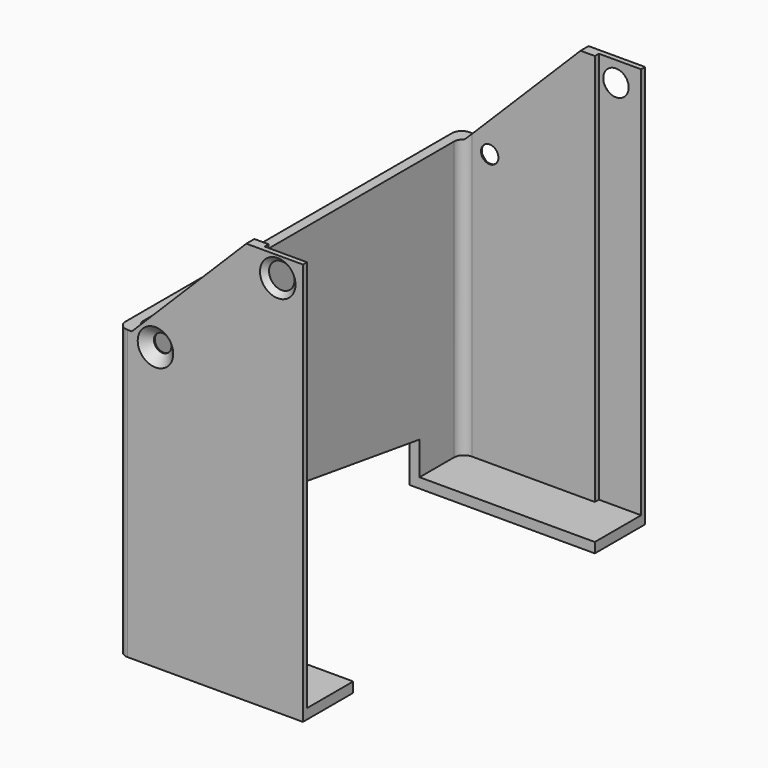
from build123d import *

# Parameters (mm, degrees)
F1_DEPTH       = 107.95
F2_T           = 2.54
F4_R           = 2.54
F3_W           = 32.7291795984
F3_H           = 105.41
F5_DEPTH       = 99.06
F7_D           = 4.4
F7_DEPTH       = 37.1856
F7_CSINK_D     = 8.96
F7_CSINK_ANGLE = 90
F7_TIP         = 1.3218933619
F9_D           = 4.4
F9_DEPTH       = 37.1856
F9_CSINK_D     = 8.96
F9_CSINK_ANGLE = 90
F9_TIP         = 1.3218933619
F10_W          = 76.2
F10_H          = 10.922
F11_DEPTH      = 56.134
F12_TEXT_SIZE  = 17.6388888889
F13_DEPTH      = 0.5334
F14_W          = 15.1848194814
F14_H          = 102.87
F15_DEPTH      = 70.1687200073
F16_DEPTH      = 70.1687200073
F17_R          = 2.54


# Not quite as in the source:
# - a shell that OpenCascade refuses in one call is made with other operations: the cavity is built on its own and cut out
# - a feature names something its author has since deleted; it is built from what else it names
# - Text() gives the source's letters only with a copy of the font that has no kerning and outlines rounded to 1/6400 em; it was checked with that copy


with BuildPart() as f1:
    # F0 (on Front) → F1 (new body)
    with BuildSketch(Plane.XZ):
        Polygon((0, 0), (0, 101.6), (-14.27734, 101.6), (-43.1686199927, 72.7087200073), (-46.7614, 72.7087200073), (-46.7614, 0), align=None)
    extrude(amount=F1_DEPTH)

    # F2: shell of thickness 2.54, made by hand


with BuildPart() as f2_core1:
    # F2_t2: copy of F1
    add(f1.part)

    # the walls: a layer under each face that stays
    f2_faces = [f2_core1.faces().sort_by_distance(p)[0] for p in [
        (-44.9650099964, -53.975, 72.7087200073),
        (-46.7614, -53.975, 36.3543600036),
        (-23.3807, -53.975, 0),
        (-23.3807, 0, 50.8),
        (-23.3807, -107.95, 50.8),
    ]]
    thicken(f2_faces, amount=-F2_T, mode=Mode.SUBTRACT)


with BuildPart() as f1_1:
    add(f1.part)

    # what is left inside the walls is the cavity
    f2_cavity = [f2_core1.part.solids().sort_by_distance(p)[0] for p in [
        (-0.0254, -71.12, 52.07),
    ]]
    add(f2_cavity, mode=Mode.SUBTRACT)

    # F4
    f4_edges = [f1_1.edges().sort_by_distance(p)[0] for p in [
        (-46.7614, -107.95, 36.35436),
        (-46.7614, 0, 36.35436),
    ]]
    fillet(f4_edges, radius=F4_R)

    # F3 (on face) → F5 (cut, through all)
    with BuildSketch(Plane.XY.offset(101.6)):
        with Locations((5.6965897992, -53.975)):
            Rectangle(F3_W, F3_H)
    extrude(amount=-F5_DEPTH, mode=Mode.SUBTRACT)

    # F7
    with Locations(Plane.XZ.offset(107.95)):
        with Locations((-37.20084, 71.12), (-6.35, 96.52)):
            CounterSinkHole(F7_D / 2, F7_CSINK_D / 2, depth=F7_DEPTH, counter_sink_angle=F7_CSINK_ANGLE)
            with Locations((0, 0, -(F7_DEPTH + F7_TIP / 2))):  # 118° drill point
                Cone(0, F7_D / 2, F7_TIP, mode=Mode.SUBTRACT)

    # F9
    with Locations(Plane(origin=(0, 0, 0), x_dir=(-1, 0, 0), z_dir=(0, 1, 0))):
        with Locations((37.20084, 71.12), (6.35, 96.52)):
            CounterSinkHole(F9_D / 2, F9_CSINK_D / 2, depth=F9_DEPTH, counter_sink_angle=F9_CSINK_ANGLE)
            with Locations((0, 0, -(F9_DEPTH + F9_TIP / 2))):  # 118° drill point
                Cone(0, F9_D / 2, F9_TIP, mode=Mode.SUBTRACT)

    # F10 (on face) → F11 (cut)
    with BuildSketch(Plane(origin=(-46.7614, 0, 0), x_dir=(0, -1, 0), z_dir=(-1, 0, 0))):
        Polygon((53.975, 16.51), (15.875, 10.922), (92.075, 10.922), align=None)
        with Locations((53.975, 5.461)):
            Rectangle(F10_W, F10_H)
    extrude(amount=-F11_DEPTH, mode=Mode.SUBTRACT)

    # F12 (on face) → F13 (cut)
    with BuildSketch(Plane(origin=(-46.7614, 0, 0), x_dir=(0, -1, 0), z_dir=(-1, 0, 0))):
        with Locations((36.2382703993, 53.6587200073)):
            Text('THC', F12_TEXT_SIZE, font='Open Sans', font_style=FontStyle.BOLD, text_align=(TextAlign.LEFT, TextAlign.BOTTOM))
        with Locations((12.3155273438, 38.4187200073)):
            Text('MACHINES', F12_TEXT_SIZE, font='Open Sans', font_style=FontStyle.ITALIC, text_align=(TextAlign.LEFT, TextAlign.BOTTOM))
    extrude(amount=-F13_DEPTH, mode=Mode.SUBTRACT)

    # F14 (on face) → F15 (cut, through all)
    with BuildSketch(Plane.XY.offset(72.7087200073)):
        with Locations((-36.6289902593, -53.975)):
            Rectangle(F14_W, F14_H)
    extrude(amount=-F15_DEPTH, mode=Mode.SUBTRACT)

    # F14 (on face) → F16 (cut, through all)
    with BuildSketch(Plane.XY.offset(72.7087200073)):
        with Locations((-36.6289902593, -53.975)):
            Rectangle(F14_W, F14_H)
    extrude(amount=-F16_DEPTH, mode=Mode.SUBTRACT)

    # F17
    f17_edges = [f1_1.edges().sort_by_distance(p)[0] for p in [
        (-44.2214, -2.54, 37.62436),
        (-44.2214, -105.41, 37.62436),
    ]]
    fillet(f17_edges, radius=F17_R)


solid = f1_1.part
